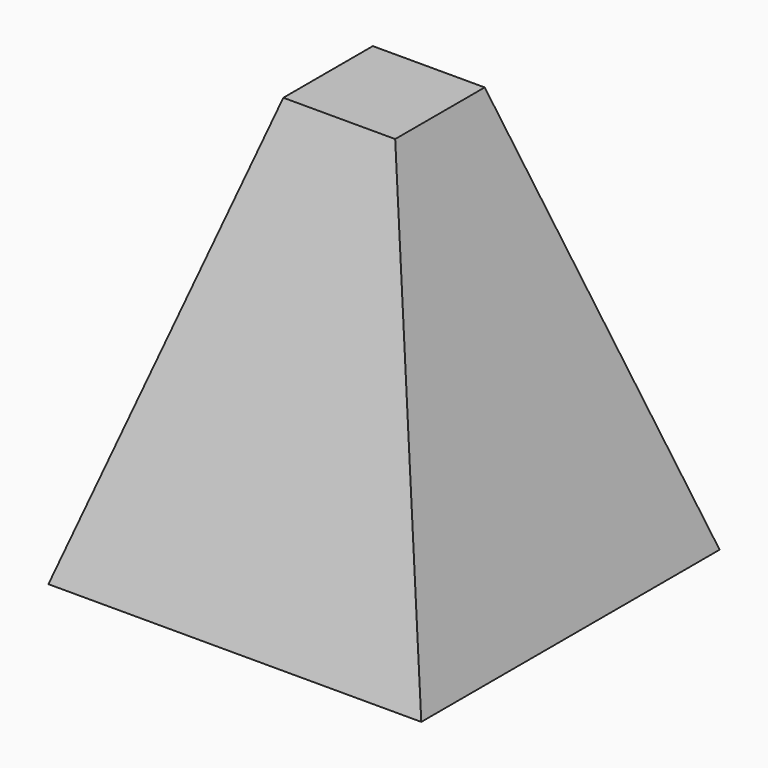
from build123d import *

# Parameters (mm, degrees)
F1_DEPTH = 25
F2_SIZE2 = 55.99999
F2_SIZE  = 17.49999


# Not quite as in the source:
# - a fillet or chamfer is up to 0.001 mm smaller than in the source, because OpenCascade refuses the exact size


with BuildPart() as f1:
    # F0 (on Front) → F1 (new body, symmetric)
    with BuildSketch(Plane.XZ):
        Polygon((25, -29.9881670944), (7.5, 26.0118329056), (-7.5, 26.0118329056), (-25, -29.9881670944), align=None)
    extrude(amount=F1_DEPTH, both=True)

    # F2 (size 17.5 and 56 in the source; OpenCascade refuses exactly that, so slightly less here)
    f2_edges = [f1.edges().sort_by_distance(p)[0] for p in [
        (0, 25, 26.011833),
        (0, -25, 26.011833),
    ]]
    f2_side = f1.faces().sort_by_distance((0, 0, 26.011833))[0]
    chamfer(f2_edges, length=F2_SIZE, length2=F2_SIZE2, reference=f2_side)


solid = f1.part
